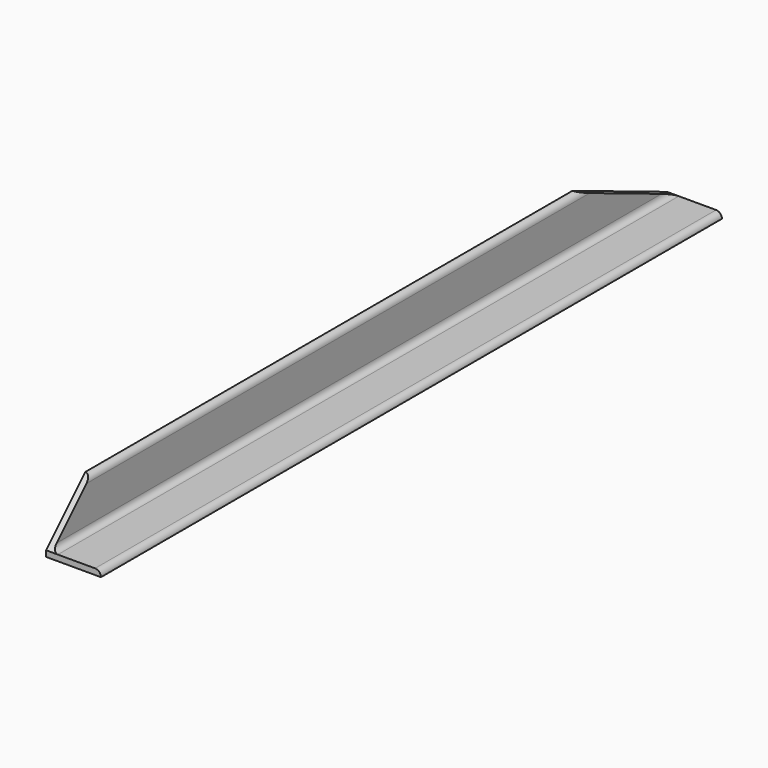
from build123d import *

# Parameters (mm, degrees)
F1_DEPTH = 628.65
F2_R     = 4.76249
F4_DEPTH = 25.4


# Not quite as in the source:
# - a fillet or chamfer is up to 0.001 mm smaller than in the source, because OpenCascade refuses the exact size


with BuildPart() as f1:
    # F0 (on Front) → F1 (new body)
    with BuildSketch(Plane.XZ):
        Polygon((0, 44.45), (0, 0), (44.45, 0), (44.45, 4.7625), (4.7625, 4.7625), (4.7625, 44.45), align=None)
    extrude(amount=F1_DEPTH)

    # F2 (radius 4.7625 in the source; OpenCascade refuses exactly that, so slightly less here)
    f2_edges = [f1.edges().sort_by_distance(p)[0] for p in [
        (4.7625, -314.325, 4.7625),
        (4.7625, -314.325, 44.45),
        (44.45, -314.325, 4.7625),
    ]]
    fillet(f2_edges, radius=F2_R)

    # F3 (on face) → F4 (cut)
    with BuildSketch(Plane(origin=(0, 0, 0), x_dir=(0, -1, 0), z_dir=(-1, 0, 0))):
        Polygon((0, 44.45), (0, 4.7625), (95.8141007567, 44.45), align=None)
        Polygon((628.65, 44.45), (588.9625, 44.45), (628.65, 4.7625), align=None)
    extrude(amount=-F4_DEPTH, mode=Mode.SUBTRACT)


solid = f1.part
